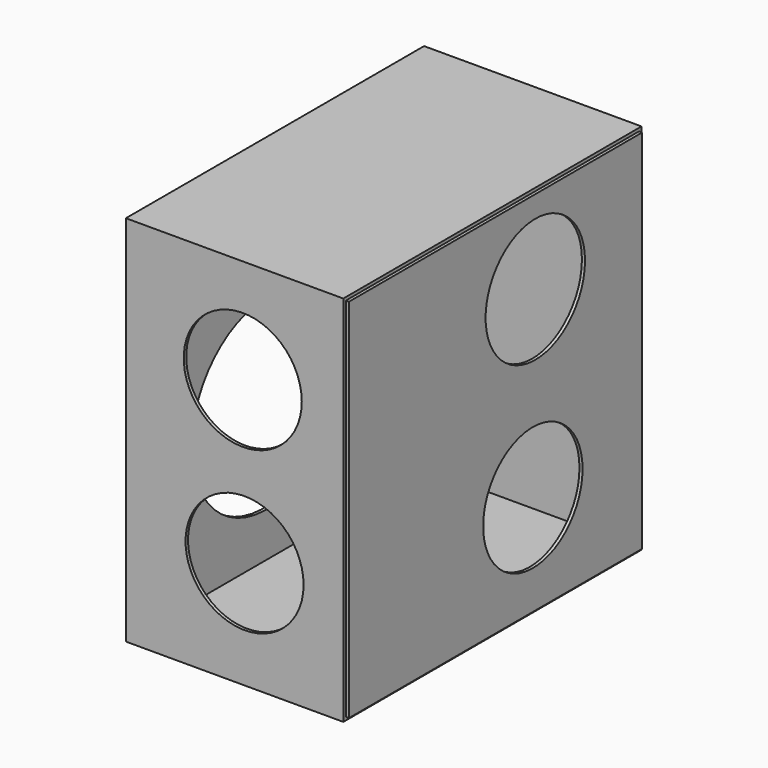
from build123d import *

# Parameters (mm, degrees)
F0_W      = 600
F0_H      = 600
F0_W_2    = 590.0000002235
F0_H_2    = 590.0000002235
F1_DEPTH  = 350
F2_DEPTH  = 5
F3_R      = 150
F4_DEPTH  = 25
F5_R      = 95
F6_DEPTH  = 25
F7_W      = 590.0000002235
F7_H      = 590.0000002235
F8_DEPTH  = 5
F12_R     = 100
F13_DEPTH = 25


# Not quite as in the source:
# - a feature names something its author has since deleted; it is built from what else it names
# - the program builds the solid bodies; features that only make, move or delete a surface that nothing else refers to are left out


with BuildPart() as f1:
    # F0 (on Right) → F1 (new body)
    with BuildSketch(Plane.YZ):
        with Locations((300, -300)):
            Rectangle(F0_W, F0_H)
        with Locations((300, -300)):
            Rectangle(F0_W_2, F0_H_2, mode=Mode.SUBTRACT)
    extrude(amount=F1_DEPTH)

    # F0 (on Right) → F2 (join)
    with BuildSketch(Plane.YZ):
        with Locations((300, -300)):
            Rectangle(F0_W_2, F0_H_2)
    extrude(amount=F2_DEPTH)

    # F3 (on face) → F4 (cut)
    with BuildSketch(Plane.YZ.offset(5)):
        with Locations((276.1940956116, -373.5814094543)):
            Circle(F3_R)
    extrude(amount=-F4_DEPTH, mode=Mode.SUBTRACT)

    # F5 (on face) → F6 (cut)
    with BuildSketch(Plane.XZ):
        with Locations((191.0568624735, -426.7022567097)):
            Circle(F5_R)
        with Locations((188.1135240477, -167.9845607586)):
            Circle(F5_R)
    extrude(amount=-F6_DEPTH, mode=Mode.SUBTRACT)


with BuildPart() as f8:
    # F7 (on face) → F8 (new body)
    with BuildSketch(Plane.YZ.offset(350)):
        with Locations((300, -300)):
            Rectangle(F7_W, F7_H)
    extrude(amount=F8_DEPTH)

    # F12 (on face) → F13 (cut)
    with BuildSketch(Plane.YZ.offset(355)):
        with Locations((380.0676831018, -139.7812012694)):
            Circle(F12_R)
        with Locations((375.1550018787, -432.9461210735)):
            Circle(F12_R)
    extrude(amount=-F13_DEPTH, mode=Mode.SUBTRACT)


solid = Compound([f1.part, f8.part])
